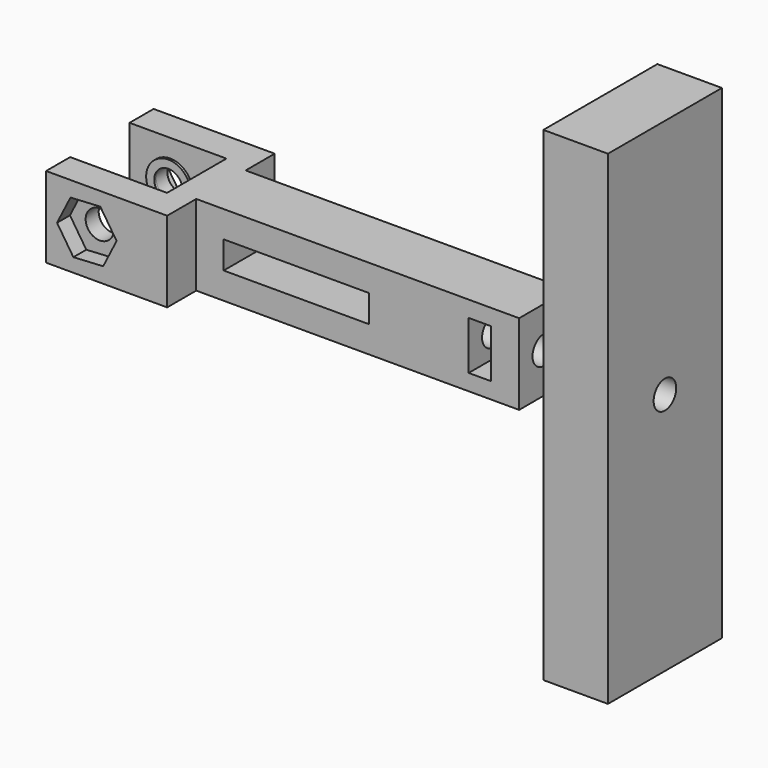
from build123d import *

# Parameters (mm, degrees)
F0_W      = 40
F0_H      = 3.825
F1_DEPTH  = 10
F2_R      = 1.75
F3_DEPTH  = 16.651
F4_W      = 18
F4_H      = 3.4
F4_W_2    = 2.75
F4_H_2    = 6
F5_DEPTH  = 12.151
F6_R      = 1.75
F7_DEPTH  = 15
F10_DEPTH = 2
F11_W     = 17.65
F11_H     = 60
F12_DEPTH = 8
F13_R     = 1.75
F14_DEPTH = 70.001
F15_R     = 2.75
F15_R_2   = 1.75
F16_DEPTH = 0.3
F17_R     = 1.75
F18_DEPTH = 2
F19_R     = 4
F20_DEPTH = 6.5


# Not quite as in the source:
# - a pattern or mirror of a feature is missing from the dataset's text; its kind, count and spacing are read off the source's solid


with BuildPart() as f1:
    # F0 (on Top) → F1 (new body)
    with BuildSketch(Plane.XY):
        Polygon((0, -3.825), (0, 0), (-3, 0), (-3, -4.6), (-15, -4.6), (-15, -8.325), (0, -8.325), align=None)
        Polygon((-3, 0), (0, 0), (0, 3.825), (0, 8.325), (-15, 8.325), (-15, 4.6), (-3, 4.6), align=None)
        with Locations((20, 1.9125)):
            Rectangle(F0_W, F0_H)
        with Locations((20, -1.9125)):
            Rectangle(F0_W, F0_H)
    extrude(amount=F1_DEPTH)

    # F2 (on face) → F3 (cut, through all)
    with BuildSketch(Plane.XZ.offset(8.325)):
        with Locations((-9.9527407438, 5)):
            Circle(F2_R)
    extrude(amount=-F3_DEPTH, mode=Mode.SUBTRACT)

    # F4 (on face) → F5 (cut, through all)
    with BuildSketch(Plane.XZ.offset(3.825)):
        with Locations((12.4002694301, 5)):
            Rectangle(F4_W, F4_H)
        with Locations((35.125, 5)):
            Rectangle(F4_W_2, F4_H_2)
    extrude(amount=-F5_DEPTH, mode=Mode.SUBTRACT)

    # F6 (on face) → F7 (cut)
    with BuildSketch(Plane.YZ.offset(40)):
        with Locations((0, 5)):
            Circle(F6_R)
    extrude(amount=-F7_DEPTH, mode=Mode.SUBTRACT)

    # F15 (on face) → F16 (join)
    with BuildSketch(Plane.XZ.offset(-4.6)):
        with Locations((-9.9527407438, 5)):
            Circle(F15_R)
        with Locations((-9.9527407438, 5)):
            Circle(F15_R_2, mode=Mode.SUBTRACT)
    f16 = extrude(amount=F16_DEPTH)

    # F16_copies: F16 across plane
    add(f16.mirror(Plane(origin=(0, 0, 0), x_dir=(0, 0, -1), z_dir=(0, -1, 0))))

    # F17 (on face) → F18 (cut)
    with BuildSketch(Plane.XZ.offset(8.325)):
        Polygon((-7.9284293953, 1.9088033227), (-6.2635302189, 5.2075067143), (-8.2878415673, 8.2987033916), (-11.9770520922, 8.0911966773), (-13.6419512686, 4.7924932857), (-11.6176399202, 1.7012966084), align=None)
        with Locations((-9.9527407438, 5)):
            Circle(F17_R, mode=Mode.SUBTRACT)
    f18 = extrude(amount=-F18_DEPTH, mode=Mode.SUBTRACT)

    # F18_copies: F18 across plane
    add(f18.mirror(Plane.ZX), mode=Mode.SUBTRACT)


with BuildPart() as f10:
    # F9 (on offset) → F10 (new body)
    with BuildSketch(Plane.YZ.offset(45)):
        Polygon((3.825, 0), (3.825, 10), (3.825, 19.8484882712), (-3.825, 19.8484882712), (-3.825, 10), (-3.825, 0), (-3.825, -10.1515117288), (3.825, -10.1515117288), align=None)
    extrude(amount=F10_DEPTH)

    # F11 (on face) → F12 (join)
    with BuildSketch(Plane.YZ.offset(47)):
        with Locations((0, 4.8484882712)):
            Rectangle(F11_W, F11_H)
    extrude(amount=F12_DEPTH)

    # F13 (on face) → F14 (cut, through all)
    with BuildSketch(Plane.YZ.offset(55)):
        with Locations((0, 5)):
            Circle(F13_R)
    extrude(amount=-F14_DEPTH, mode=Mode.SUBTRACT)

    # F19 (on face) → F20 (cut)
    with BuildSketch(Plane(origin=(47, 0, 0), x_dir=(0, -1, 0), z_dir=(-1, 0, 0))):
        with Locations((0, 28)):
            Circle(F19_R)
        with Locations((0, -18)):
            Circle(F19_R)
    extrude(amount=-F20_DEPTH, mode=Mode.SUBTRACT)


solid = Compound([f1.part, f10.part])
